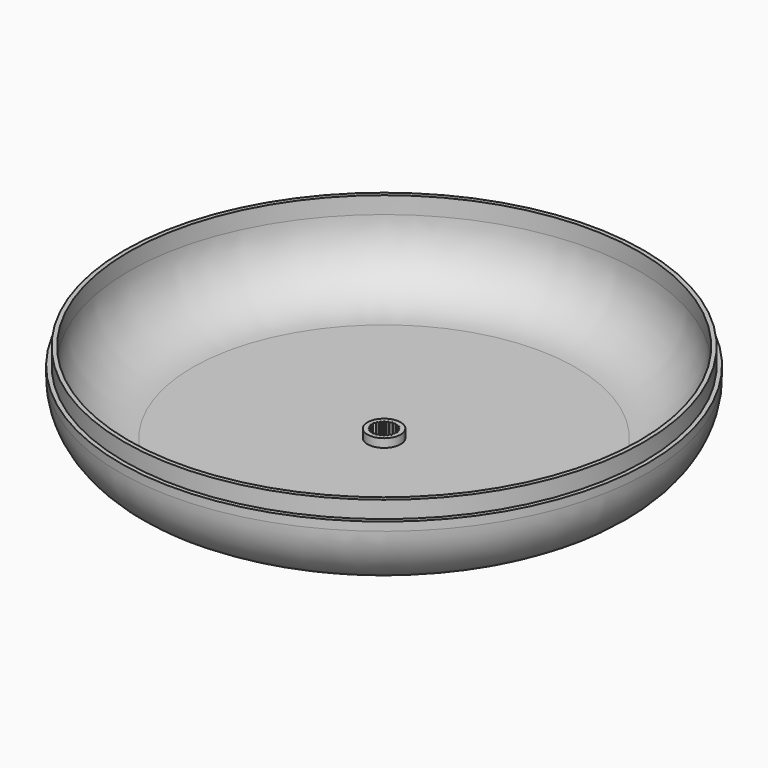
from build123d import *

# Parameters (mm, degrees)
F0_R     = 62
F1_DEPTH = 17
F2_R     = 60
F3_DEPTH = 15
F4_R     = 14.99999
F5_R     = 61
F5_R_2   = 60
F6_DEPTH = 4
F7_R     = 3.9
F8_DEPTH = 2
F9_DEPTH = 1
F10_D    = 3


# Not quite as in the source:
# - a fillet or chamfer is up to 0.001 mm smaller than in the source, because OpenCascade refuses the exact size


with BuildPart() as f1:
    # F0 (on Top) → F1 (new body)
    with BuildSketch(Plane.XY):
        Circle(F0_R)
    extrude(amount=-F1_DEPTH)

    # F2 (on face) → F3 (cut)
    with BuildSketch(Plane.XY):
        Circle(F2_R)
    extrude(amount=-F3_DEPTH, mode=Mode.SUBTRACT)

    # F4 (radius 15 in the source; OpenCascade refuses exactly that, so slightly less here)
    f4_edges = [f1.edges().sort_by_distance(p)[0] for p in [
        (-60, 0, -15),
        (-62, 0, -17),
    ]]
    fillet(f4_edges, radius=F4_R)

    # F5 (on face) → F6 (join)
    with BuildSketch(Plane.XY):
        Circle(F5_R)
        Circle(F5_R_2, mode=Mode.SUBTRACT)
    extrude(amount=F6_DEPTH)

    # F7 (on face) → F8 (join)
    with BuildSketch(Plane.XY.offset(-15)):
        Circle(F7_R)
        with BuildLine():
            ThreePointArc((2.6792506443, 1.1097819539), (2.8011848962, 0.7505752308), (2.875190098, 0.3785259574))
            ThreePointArc((2.875190098, 0.3785259574), (2.8937908774, 0.1896690748), (2.9, 0))
            ThreePointArc((2.9, 0), (2.8937908774, -0.1896690748), (2.875190098, -0.3785259574))
            ThreePointArc((2.875190098, -0.3785259574), (2.8011848962, -0.7505752308), (2.6792506443, -1.1097819539))
            ThreePointArc((2.6792506443, -1.1097819539), (2.511473671, -1.45), (2.3007246868, -1.7654081441))
            ThreePointArc((2.3007246868, -1.7654081441), (2.0506096654, -2.0506096654), (1.7654081441, -2.3007246868))
            ThreePointArc((1.7654081441, -2.3007246868), (1.45, -2.511473671), (1.1097819539, -2.6792506443))
            ThreePointArc((1.1097819539, -2.6792506443), (0.7505752308, -2.8011848962), (0.3785259574, -2.875190098))
            ThreePointArc((0.3785259574, -2.875190098), (0, -2.9), (-0.3785259574, -2.875190098))
            ThreePointArc((-0.3785259574, -2.875190098), (-0.7505752308, -2.8011848962), (-1.1097819539, -2.6792506443))
            ThreePointArc((-1.1097819539, -2.6792506443), (-1.45, -2.511473671), (-1.7654081441, -2.3007246868))
            ThreePointArc((-1.7654081441, -2.3007246868), (-2.0506096654, -2.0506096654), (-2.3007246868, -1.7654081441))
            ThreePointArc((-2.3007246868, -1.7654081441), (-2.511473671, -1.45), (-2.6792506443, -1.1097819539))
            ThreePointArc((-2.6792506443, -1.1097819539), (-2.8011848962, -0.7505752308), (-2.875190098, -0.3785259574))
            ThreePointArc((-2.875190098, -0.3785259574), (-2.9, 0), (-2.875190098, 0.3785259574))
            ThreePointArc((-2.875190098, 0.3785259574), (-2.8011848962, 0.7505752308), (-2.6792506443, 1.1097819539))
            ThreePointArc((-2.6792506443, 1.1097819539), (-2.511473671, 1.45), (-2.3007246868, 1.7654081441))
            ThreePointArc((-2.3007246868, 1.7654081441), (-2.0506096654, 2.0506096654), (-1.7654081441, 2.3007246868))
            ThreePointArc((-1.7654081441, 2.3007246868), (-1.45, 2.511473671), (-1.1097819539, 2.6792506443))
            ThreePointArc((-1.1097819539, 2.6792506443), (-0.7505752308, 2.8011848962), (-0.3785259574, 2.875190098))
            ThreePointArc((-0.3785259574, 2.875190098), (0, 2.9), (0.3785259574, 2.875190098))
            ThreePointArc((0.3785259574, 2.875190098), (0.7505752308, 2.8011848962), (1.1097819539, 2.6792506443))
            ThreePointArc((1.1097819539, 2.6792506443), (1.45, 2.511473671), (1.7654081441, 2.3007246868))
            ThreePointArc((1.7654081441, 2.3007246868), (2.0506096654, 2.0506096654), (2.3007246868, 1.7654081441))
            ThreePointArc((2.3007246868, 1.7654081441), (2.511473671, 1.45), (2.6792506443, 1.1097819539))
        make_face(mode=Mode.SUBTRACT)
        with BuildLine():
            Line((-2.6792506443, 1.1097819539), (-2.2170250337, 1.28))
            Line((-2.2170250337, 1.28), (-2.3007246868, 1.7654081441))
            ThreePointArc((-2.3007246868, 1.7654081441), (-2.511473671, 1.45), (-2.6792506443, 1.1097819539))
        make_face()
        with BuildLine():
            Line((-2.3007246868, 1.7654081441), (-1.8101933598, 1.8101933598))
            Line((-1.8101933598, 1.8101933598), (-1.7654081441, 2.3007246868))
            ThreePointArc((-1.7654081441, 2.3007246868), (-2.0506096654, 2.0506096654), (-2.3007246868, 1.7654081441))
        make_face()
        with BuildLine():
            Line((-1.7654081441, 2.3007246868), (-1.28, 2.2170250337))
            Line((-1.28, 2.2170250337), (-1.1097819539, 2.6792506443))
            ThreePointArc((-1.1097819539, 2.6792506443), (-1.45, 2.511473671), (-1.7654081441, 2.3007246868))
        make_face()
        with BuildLine():
            Line((-1.1097819539, 2.6792506443), (-0.6625767555, 2.4727701153))
            Line((-0.6625767555, 2.4727701153), (-0.3785259574, 2.875190098))
            ThreePointArc((-0.3785259574, 2.875190098), (-0.7505752308, 2.8011848962), (-1.1097819539, 2.6792506443))
        make_face()
        with BuildLine():
            Line((-0.3785259574, 2.875190098), (0, 2.56))
            Line((0, 2.56), (0.3785259574, 2.875190098))
            ThreePointArc((0.3785259574, 2.875190098), (0, 2.9), (-0.3785259574, 2.875190098))
        make_face()
        with BuildLine():
            Line((0.3785259574, 2.875190098), (0.6625767555, 2.4727701153))
            Line((0.6625767555, 2.4727701153), (1.1097819539, 2.6792506443))
            ThreePointArc((1.1097819539, 2.6792506443), (0.7505752308, 2.8011848962), (0.3785259574, 2.875190098))
        make_face()
        with BuildLine():
            Line((1.1097819539, 2.6792506443), (1.28, 2.2170250337))
            Line((1.28, 2.2170250337), (1.7654081441, 2.3007246868))
            ThreePointArc((1.7654081441, 2.3007246868), (1.45, 2.511473671), (1.1097819539, 2.6792506443))
        make_face()
        with BuildLine():
            Line((1.7654081441, 2.3007246868), (1.8101933598, 1.8101933598))
            Line((1.8101933598, 1.8101933598), (2.3007246868, 1.7654081441))
            ThreePointArc((2.3007246868, 1.7654081441), (2.0506096654, 2.0506096654), (1.7654081441, 2.3007246868))
        make_face()
        with BuildLine():
            Line((2.3007246868, 1.7654081441), (2.2170250337, 1.28))
            Line((2.2170250337, 1.28), (2.6792506443, 1.1097819539))
            ThreePointArc((2.6792506443, 1.1097819539), (2.511473671, 1.45), (2.3007246868, 1.7654081441))
        make_face()
        with BuildLine():
            Line((2.6792506443, 1.1097819539), (2.4727701153, 0.6625767555))
            Line((2.4727701153, 0.6625767555), (2.875190098, 0.3785259574))
            ThreePointArc((2.875190098, 0.3785259574), (2.8011848962, 0.7505752308), (2.6792506443, 1.1097819539))
        make_face()
        with BuildLine():
            ThreePointArc((2.9, 0), (2.8937908774, 0.1896690748), (2.875190098, 0.3785259574))
            Line((2.875190098, 0.3785259574), (2.56, 0))
            Line((2.56, 0), (2.875190098, -0.3785259574))
            ThreePointArc((2.875190098, -0.3785259574), (2.8937908774, -0.1896690748), (2.9, 0))
        make_face()
        with BuildLine():
            Line((2.875190098, -0.3785259574), (2.4727701153, -0.6625767555))
            Line((2.4727701153, -0.6625767555), (2.6792506443, -1.1097819539))
            ThreePointArc((2.6792506443, -1.1097819539), (2.8011848962, -0.7505752308), (2.875190098, -0.3785259574))
        make_face()
        with BuildLine():
            Line((2.6792506443, -1.1097819539), (2.2170250337, -1.28))
            Line((2.2170250337, -1.28), (2.3007246868, -1.7654081441))
            ThreePointArc((2.3007246868, -1.7654081441), (2.511473671, -1.45), (2.6792506443, -1.1097819539))
        make_face()
        with BuildLine():
            Line((2.3007246868, -1.7654081441), (1.8101933598, -1.8101933598))
            Line((1.8101933598, -1.8101933598), (1.7654081441, -2.3007246868))
            ThreePointArc((1.7654081441, -2.3007246868), (2.0506096654, -2.0506096654), (2.3007246868, -1.7654081441))
        make_face()
        with BuildLine():
            Line((1.7654081441, -2.3007246868), (1.28, -2.2170250337))
            Line((1.28, -2.2170250337), (1.1097819539, -2.6792506443))
            ThreePointArc((1.1097819539, -2.6792506443), (1.45, -2.511473671), (1.7654081441, -2.3007246868))
        make_face()
        with BuildLine():
            Line((-2.875190098, 0.3785259574), (-2.4727701153, 0.6625767555))
            Line((-2.4727701153, 0.6625767555), (-2.6792506443, 1.1097819539))
            ThreePointArc((-2.6792506443, 1.1097819539), (-2.8011848962, 0.7505752308), (-2.875190098, 0.3785259574))
        make_face()
        with BuildLine():
            Line((-2.875190098, -0.3785259574), (-2.56, 0))
            Line((-2.56, 0), (-2.875190098, 0.3785259574))
            ThreePointArc((-2.875190098, 0.3785259574), (-2.9, 0), (-2.875190098, -0.3785259574))
        make_face()
        with BuildLine():
            Line((-2.6792506443, -1.1097819539), (-2.4727701153, -0.6625767555))
            Line((-2.4727701153, -0.6625767555), (-2.875190098, -0.3785259574))
            ThreePointArc((-2.875190098, -0.3785259574), (-2.8011848962, -0.7505752308), (-2.6792506443, -1.1097819539))
        make_face()
        with BuildLine():
            Line((-2.3007246868, -1.7654081441), (-2.2170250337, -1.28))
            Line((-2.2170250337, -1.28), (-2.6792506443, -1.1097819539))
            ThreePointArc((-2.6792506443, -1.1097819539), (-2.511473671, -1.45), (-2.3007246868, -1.7654081441))
        make_face()
        with BuildLine():
            Line((-1.7654081441, -2.3007246868), (-1.8101933598, -1.8101933598))
            Line((-1.8101933598, -1.8101933598), (-2.3007246868, -1.7654081441))
            ThreePointArc((-2.3007246868, -1.7654081441), (-2.0506096654, -2.0506096654), (-1.7654081441, -2.3007246868))
        make_face()
        with BuildLine():
            Line((-1.1097819539, -2.6792506443), (-1.28, -2.2170250337))
            Line((-1.28, -2.2170250337), (-1.7654081441, -2.3007246868))
            ThreePointArc((-1.7654081441, -2.3007246868), (-1.45, -2.511473671), (-1.1097819539, -2.6792506443))
        make_face()
        with BuildLine():
            Line((-0.3785259574, -2.875190098), (-0.6625767555, -2.4727701153))
            Line((-0.6625767555, -2.4727701153), (-1.1097819539, -2.6792506443))
            ThreePointArc((-1.1097819539, -2.6792506443), (-0.7505752308, -2.8011848962), (-0.3785259574, -2.875190098))
        make_face()
        with BuildLine():
            Line((0.3785259574, -2.875190098), (0, -2.56))
            Line((0, -2.56), (-0.3785259574, -2.875190098))
            ThreePointArc((-0.3785259574, -2.875190098), (0, -2.9), (0.3785259574, -2.875190098))
        make_face()
        with BuildLine():
            Line((1.1097819539, -2.6792506443), (0.6625767555, -2.4727701153))
            Line((0.6625767555, -2.4727701153), (0.3785259574, -2.875190098))
            ThreePointArc((0.3785259574, -2.875190098), (0.7505752308, -2.8011848962), (1.1097819539, -2.6792506443))
        make_face()
    extrude(amount=F8_DEPTH)

    # F9 (cut): a face of the model
    f9_faces = [f1.faces().sort_by_distance(p)[0] for p in [
        (0, 0, -15),
    ]]
    extrude(f9_faces, amount=-F9_DEPTH, mode=Mode.SUBTRACT)

    # F10 (through all)
    with Locations(Plane.XY.offset(-15)):
        with Locations((0, 0)):
            Hole(F10_D / 2)


solid = f1.part
